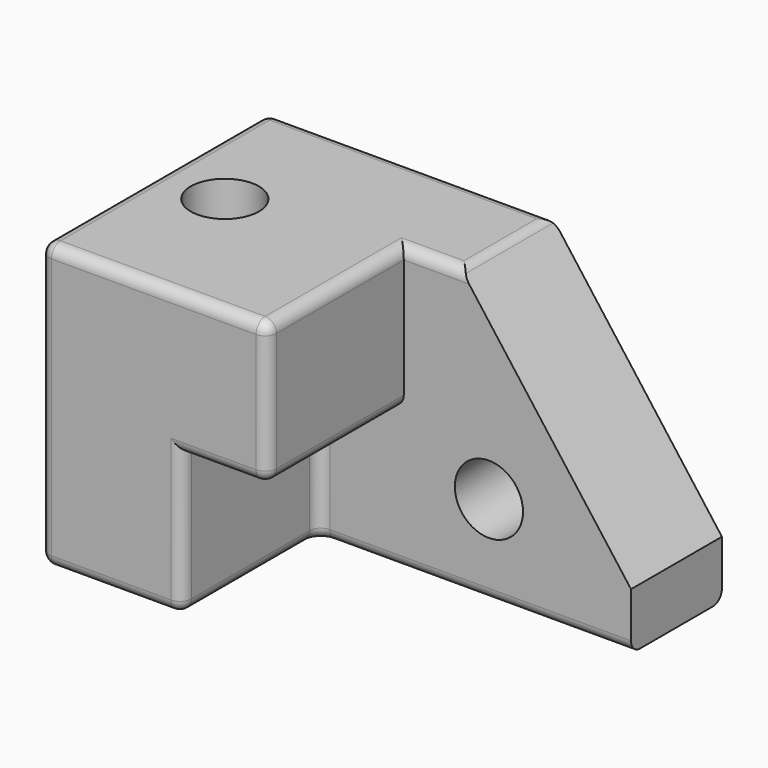
from build123d import *

# Parameters (mm, degrees)
F0_W     = 203.2
F0_H     = 127
F1_DEPTH = 127
F3_DEPTH = 76.2
F4_SIZE2 = 101.6
F4_SIZE  = 76.2
F5_R     = 5.08
F6_R     = 15.24
F7_DEPTH = 50.8
F8_R     = 15.24
F9_DEPTH = 127


with BuildPart() as f1:
    # F0 (on Front) → F1 (new body)
    with BuildSketch(Plane.XZ):
        with Locations((-21.9353889487, -0.1176632941)):
            Rectangle(F0_W, F0_H)
    extrude(amount=F1_DEPTH)

    # F2 (on face) → F3 (cut)
    with BuildSketch(Plane.XZ.offset(127)):
        Polygon((79.6646110513, 63.3823367059), (-21.9353889487, 63.3823367059), (-21.9353889487, 0), (-60.0353889487, 0), (-60.0353889487, -63.6176632941), (79.6646110513, -63.6176632941), align=None)
    extrude(amount=-F3_DEPTH, mode=Mode.SUBTRACT)

    # F4
    f4_edges = [f1.edges().sort_by_distance(p)[0] for p in [
        (79.664611, -25.4, 63.382337),
    ]]
    f4_side = f1.faces().sort_by_distance((-43.706818, -52.614286, 63.382337))[0]
    chamfer(f4_edges, length=F4_SIZE, length2=F4_SIZE2, reference=f4_side)

    # F5
    f5_edges = [f1.edges().sort_by_distance(p)[0] for p in [
        (-72.735389, -127, 63.382337),
        (-21.935389, -88.9, 63.382337),
        (-40.985389, -127, 0),
        (-21.935389, -88.9, 0),
        (-21.935389, -127, 31.691168),
        (-60.035389, -127, -31.808832),
        (-60.035389, -50.8, -31.808832),
        (9.814611, -50.8, -63.617663),
        (3.464611, -25.4, 63.382337),
        (-9.235389, -50.8, 63.382337),
        (-123.535389, -127, -0.117663),
        (-123.535389, 0, -0.117663),
        (-123.535389, -63.5, -63.617663),
        (-123.535389, -63.5, 63.382337),
        (-21.935389, 0, -63.617663),
        (-60.035389, 0, 63.382337),
        (-91.785389, -127, -63.617663),
        (-60.035389, -88.9, -63.617663),
    ]]
    fillet(f5_edges, radius=F5_R)

    # F6 (on face) → F7 (cut, through all)
    with BuildSketch(Plane.XZ.offset(50.8)):
        with Locations((16.1317326128, -23.4769377857)):
            Circle(F6_R)
    extrude(amount=-F7_DEPTH, mode=Mode.SUBTRACT)

    # F8 (on face) → F9 (cut, through all)
    with BuildSketch(Plane(origin=(0, 0, -63.6176632941), x_dir=(1, 0, 0), z_dir=(0, 0, -1))):
        with Locations((-93.4789702296, 61.3736882806)):
            Circle(F8_R)
    extrude(amount=-F9_DEPTH, mode=Mode.SUBTRACT)


solid = f1.part
